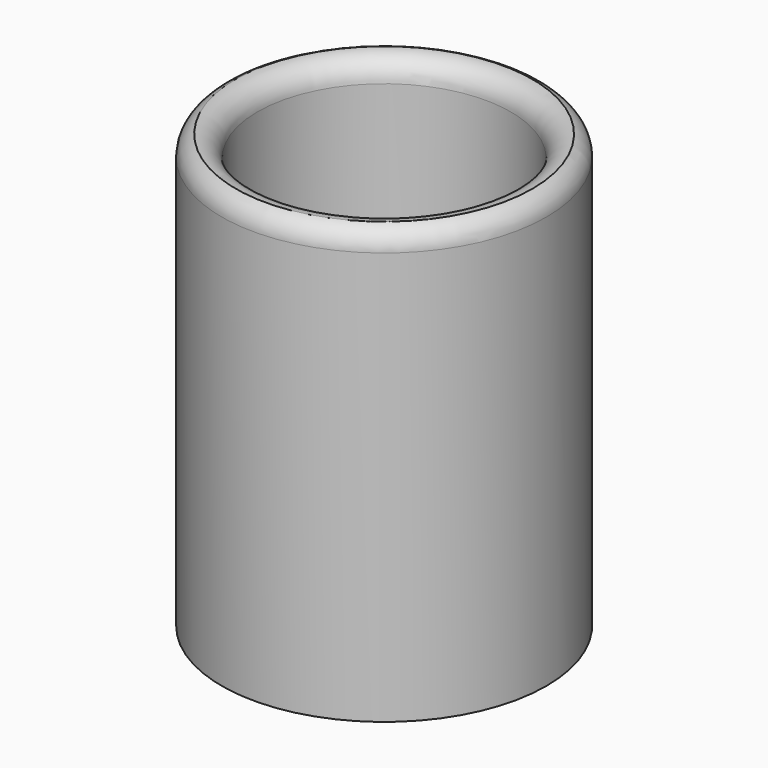
from build123d import *

# Parameters (mm, degrees)
F0_R     = 38.1
F1_DEPTH = 101.6
F2_T     = -8.382
F3_R     = 5.08


# Not quite as in the source:
# - a fillet or chamfer that OpenCascade refuses, or shapes differently, is made with other operations: its cross-section is extruded or revolved along the edge and cut away or added


with BuildPart() as f1:
    # F0 (on Top) → F1 (new body)
    with BuildSketch(Plane.XY):
        Circle(F0_R)
    extrude(amount=F1_DEPTH)

    # F2
    f2_openings = [f1.faces().sort_by_distance(p)[0] for p in [
        (0, 0, 101.6),
    ]]
    offset(amount=F2_T, openings=f2_openings)

    # F3
    f3_edges = [f1.edges().sort_by_distance(p)[0] for p in [
        (-29.718, 0, 101.6),
    ]]
    fillet(f3_edges, radius=F3_R)

    # F4: fillet of radius 5.08 on 1 edges, made by hand

    # F4_s1 → F4_t2 (revolve, cut)
    with BuildSketch(Plane.XZ):
        with BuildLine():
            ThreePointArc((34.798, 101.6), (37.1936458882, 99.737357105), (38.1, 96.8413115252))
            Line((38.1, 96.8413115252), (38.1, 101.6))
            Line((38.1, 101.6), (34.798, 101.6))
        make_face()
    revolve(axis=Axis((0, 0, 101.6), (0, 0, 1)), mode=Mode.SUBTRACT)


solid = f1.part
